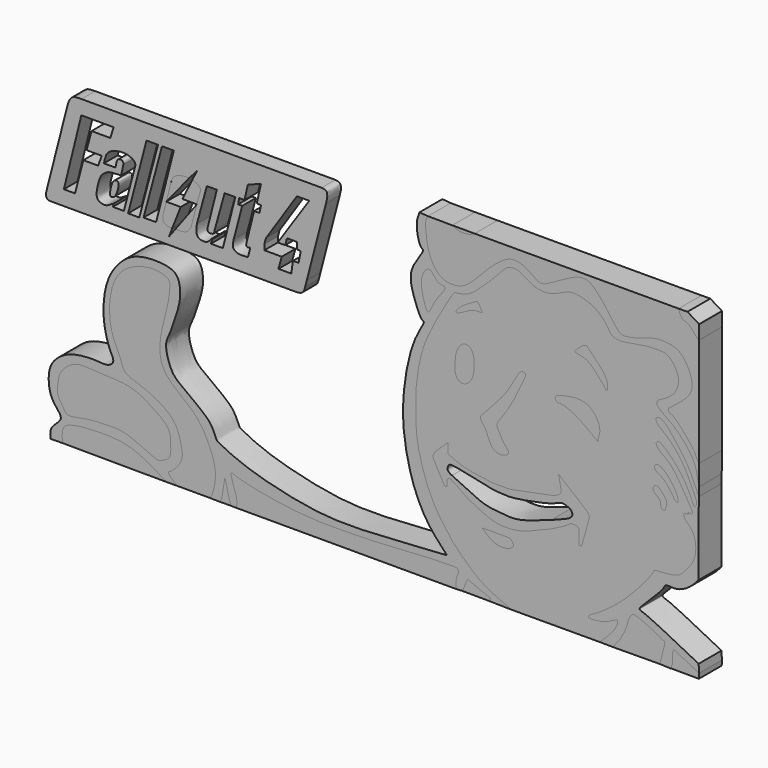
from build123d import *

# Parameters (mm, degrees)
F2_DEPTH       = 3.81
F3_DEPTH       = 50.8
F3_DEPTH_BACK  = 50.8
F4_DEPTH       = 3.81
F7_DEPTH       = 6.35
F8_DEPTH       = 6.35
F9_DEPTH       = 6.35
F10_DEPTH      = 6.35
F11_DEPTH      = 50.8
F11_DEPTH_BACK = 50.8
F12_DEPTH      = 6.35


# Not quite as in the source:
# - the program builds the solid bodies; features that only make, move or delete a surface that nothing else refers to are left out


with BuildPart() as f2:
    # F1 (on Front) → F2 (new body)
    with BuildSketch(Plane.XZ):
        with BuildLine():
            Line((-12.4136926606, 36.7652848363), (-63.8129115105, 36.7652848363))
            add(Edge.make_bspline(
                [(-66.8279528618, 34.8988324404), (-66.5930374758, 35.4970886217), (-66.1023482487, 36.7467209609), (-64.5973817053, 36.7589239674), (-63.8129115105, 36.7652848363)],
                knots=[0, 0, 0, 0, 0.478745758, 1, 1, 1, 1], degree=3))
            Line((-66.8279528618, 34.8988324404), (-71.5658739209, 16.3778848946))
            add(Edge.make_bspline(
                [(-70.5474168062, 14.5114324987), (-70.8911246373, 14.5193117419), (-71.5807384925, 14.5351206203), (-71.7483771612, 15.6377549861), (-71.6249795935, 16.1381857201), (-71.5658739209, 16.3778848946)],
                knots=[0, 0, 0, 0, 0.3411096868, 0.6844009503, 1, 1, 1, 1], degree=3))
            Line((-70.5474168062, 14.5114324987), (-68.8379779458, 14.5114324987))
            Line((-68.8379779458, 14.5114324987), (-17.2951817513, 14.5114324987))
            Line((-17.2951817513, 14.5114324987), (-15.7989468426, 14.5114324987))
            add(Edge.make_bspline(
                [(-14.0476999804, 16.1771159619), (-14.1856649693, 15.6813406422), (-14.4532535126, 14.7197648347), (-15.3598022305, 14.5794182878), (-15.7989468426, 14.5114324987)],
                knots=[0, 0, 0, 0, 0.5155863073, 1, 1, 1, 1], degree=3))
            Line((-14.0476999804, 16.1771159619), (-13.7058505788, 17.5264719874))
            Line((-13.7058505788, 17.5264719874), (-9.3986541033, 34.0373963118))
            add(Edge.make_bspline(
                [(-9.3986541033, 34.0373963118), (-9.2794631114, 34.5027471456), (-9.0568676553, 35.3718143421), (-9.2273719999, 36.6584162884), (-10.0001459599, 36.7299325533), (-10.3821475059, 36.7652848363)],
                knots=[0, 0, 0, 0, 0.3682382464, 0.6877043236, 1, 1, 1, 1], degree=3))
            Line((-10.3821475059, 36.7652848363), (-12.4136926606, 36.7652848363))
        make_face()
    extrude(amount=F2_DEPTH)

    # F0 (on Front) → F3 (cut, two sides)
    with BuildSketch(Plane.XZ) as f3_sk:
        Polygon((-56.6699653864, 33.5655286908), (-63.8487637043, 33.5655286908), (-67.7311718464, 17.8161300719), (-65.2405694127, 17.8161300719), (-63.4092465043, 24.9216724187), (-60.1128563285, 24.9216724187), (-59.3070760369, 27.119262144), (-62.6767128706, 27.119262144), (-61.5779198706, 31.2214307487), (-57.4024952948, 31.2214307487), align=None)
        Polygon((-46.7808097601, 33.3457700908), (-49.3446663022, 33.3457700908), (-53.4468330443, 17.7428778261), (-50.9562306106, 17.7428778261), align=None)
        Polygon((-43.2646647096, 33.3457700908), (-45.9017753601, 33.3457700908), (-50.0039421022, 18.0358905345), (-47.2203269601, 18.0358905345), align=None)
        with BuildLine():
            Line((-33.7026938796, 28.787843883), (-35.9268300235, 28.787843883))
            Line((-35.9268300235, 28.787843883), (-38.1369553506, 20.6729974598))
            add(Edge.make_bspline(
                [(-34.7237996757, 18.7542904168), (-34.7942705526, 18.7755190956), (-35.0111876698, 18.8408633059), (-35.483336033, 17.8389711757), (-37.0910656938, 17.5716890977), (-38.4823420582, 18.4677567251), (-38.2602498605, 19.8857810743), (-38.1369553506, 20.6729974598)],
                knots=[0, 0, 0, 0, 0.0879184805, 0.2706227618, 0.5039064203, 0.7245935905, 1, 1, 1, 1], degree=3))
            Line((-34.7237996757, 18.7542904168), (-35.0293107331, 17.7858132069))
            Line((-35.0293107331, 17.7858132069), (-32.357059703, 17.7858132069))
            Line((-32.357059703, 17.7858132069), (-29.5966751873, 28.6820493639))
            Line((-29.5966751873, 28.6820493639), (-31.9803804159, 28.6820493639))
            Line((-31.9803804159, 28.6820493639), (-34.1977849603, 20.6994023174))
            add(Edge.make_bspline(
                [(-35.7640907168, 20.6507649273), (-35.7779261817, 20.370142077), (-35.805227327, 19.8163966625), (-34.9705905732, 19.7482981395), (-34.3340216083, 19.9094108137), (-34.2448802558, 20.4263121918), (-34.1977849603, 20.6994023174)],
                knots=[0, 0, 0, 0, 0.2567288564, 0.5065960482, 0.7393240705, 1, 1, 1, 1], degree=3))
            Line((-35.7640907168, 20.6507649273), (-33.7026938796, 28.787843883))
        make_face()
        with BuildLine():
            Line((-24.8345918953, 28.9711412042), (-23.8816402853, 33.1264324486))
            Line((-23.8816402853, 33.1264324486), (-26.8109887838, 32.041490078))
            Line((-26.8109887838, 32.041490078), (-27.5433268398, 28.7866592407))
            Line((-27.5433268398, 28.7866592407), (-28.7367645651, 28.7866592407))
            Line((-28.7367645651, 28.7866592407), (-28.9596170187, 27.4700615555))
            Line((-28.9596170187, 27.4700615555), (-28.056461364, 27.4700615555))
            Line((-28.056461364, 27.4700615555), (-29.9493856728, 20.294258371))
            add(Edge.make_bspline(
                [(-29.9493856728, 20.294258371), (-30.092060965, 19.7383291905), (-30.362724298, 18.6836991804), (-29.1729702441, 17.6258337898), (-27.6673140995, 17.7559010596), (-26.7947631998, 17.8312770434)],
                knots=[0, 0, 0, 0, 0.3191430371, 0.6054329153, 1, 1, 1, 1], degree=3))
            Line((-26.7947631998, 17.8312770434), (-26.2655150145, 19.8375806212))
            add(Edge.make_bspline(
                [(-27.0875357091, 20.6291563809), (-27.1541227134, 20.2999555053), (-27.288565148, 19.6352827564), (-26.6086699315, 19.7697251909), (-26.2655150145, 19.8375806212)],
                knots=[0, 0, 0, 0, 0.4952826426, 1, 1, 1, 1], degree=3))
            Line((-27.0875357091, 20.6291563809), (-25.413049385, 27.3271016777))
            Line((-25.413049385, 27.3271016777), (-24.2256876081, 27.3271016777))
            Line((-24.2256876081, 27.3271016777), (-23.8816402853, 28.9711412042))
            Line((-23.8816402853, 28.9711412042), (-24.8345918953, 28.9711412042))
        make_face()
        Polygon((-13.1602361798, 33.3156175911), (-15.8830825239, 33.3156175911), (-22.7770470083, 22.87437208), (-23.1365542859, 21.573740989), (-23.1365542859, 20.3725714236), (-19.269622429, 20.3725714236), (-19.9958086014, 17.7583042532), (-17.1447917819, 17.7583042532), (-16.7751051486, 20.3725714236), (-15.528453514, 20.3725714236), (-15.0296529755, 22.8712726384), (-15.9237217158, 22.8712726384), (-15.9237217158, 24.3749339134), (-18.1182529777, 24.3749339134), (-18.4840094298, 22.8712726384), (-20.1502274722, 22.8712726384), align=None)
        with BuildLine():
            add(Edge.make_bspline(
                [(-56.0185929589, 26.9032054337), (-55.9315318538, 27.1764927811), (-55.7607888192, 27.7124601453), (-54.897529735, 27.8059599362), (-54.4600894732, 27.4133429295), (-54.4765988554, 27.1444736762), (-54.4841401279, 27.0216576755)],
                knots=[0, 0, 0, 0, 0.2903149552, 0.5693616728, 0.8032899767, 1, 1, 1, 1], degree=3))
            Line((-54.4841401279, 27.0216576755), (-54.9910180271, 24.6682912111))
            add(Edge.make_bspline(
                [(-56.6504810475, 18.6222402498), (-56.8782994422, 18.5027217057), (-57.3779649704, 18.2405861723), (-58.3446885415, 17.5424606272), (-59.9100095305, 17.8517225749), (-60.6532111412, 18.8562404414), (-60.1776503547, 21.2198138616), (-59.6312458469, 23.1546101881), (-58.5574681299, 24.0817746184), (-57.404840766, 24.6180593038), (-55.8833951014, 24.6497207495), (-54.9910180271, 24.6682912111)],
                knots=[0, 0, 0, 0, 0.081900036, 0.1796282728, 0.2890494758, 0.3835465603, 0.522869379, 0.6535863473, 0.7573575505, 0.8576823582, 1, 1, 1, 1], degree=3))
            Line((-56.6504810475, 18.6222402498), (-56.8375065923, 17.9108748642))
            Line((-56.8375065923, 17.9108748642), (-54.3889209023, 17.9108748642))
            Line((-54.3889209023, 17.9108748642), (-52.0221553743, 26.9130412489))
            add(Edge.make_bspline(
                [(-58.8288195431, 25.7906652987), (-58.6285272673, 26.6353679225), (-58.2807075766, 28.1022452856), (-57.0637613923, 28.814659604), (-55.5491126764, 29.2714406503), (-53.5448376569, 29.3766637698), (-51.5666326897, 28.3006651858), (-51.8813934139, 27.3418336501), (-52.0221553743, 26.9130412489)],
                knots=[0, 0, 0, 0, 0.1954333106, 0.3393818029, 0.4984152875, 0.6821298917, 0.8578475134, 1, 1, 1, 1], degree=3))
            Line((-58.8288195431, 25.7906652987), (-56.2582165003, 25.7906652987))
            Line((-56.2582165003, 25.7906652987), (-56.0185929589, 26.9032054337))
        make_face()
        with BuildLine():
            add(Edge.make_bspline(
                [(-55.7971820235, 23.2893116772), (-56.007171461, 23.4078330879), (-56.8609223877, 23.1168172963), (-57.1807348709, 21.9058389294), (-57.5572301952, 20.4756311128), (-57.4030916495, 19.5969734365), (-56.5403624052, 19.864360996), (-56.0255461327, 20.5938708576), (-55.5265065234, 22.212219434), (-55.5748715361, 23.1638360681), (-55.7971820235, 23.2893116772)],
                knots=[0, 0, 0, 0, 0.1148834001, 0.2515738645, 0.4032942387, 0.501768148, 0.600291131, 0.715809865, 0.8783758603, 1, 1, 1, 1], degree=3))
        make_face(mode=Mode.SUBTRACT)
        Polygon((-39.8514476016, 29.0725264404), (-44.9494868517, 22.7973349392), (-41.7441688478, 22.7973349392), (-43.6099198481, 18.058598945), (-43.7186323106, 17.7824851125), (-44.3634614513, 16.1313116673), (-42.8970865035, 18.0979792621), (-38.1369553506, 24.4821552187), (-41.3537174463, 24.490237236), (-39.1451600054, 28.9608438894), (-38.1369553506, 31.0016721487), (-39.7662445903, 29.1774030775), align=None)
        with BuildLine():
            Line((-43.8660690067, 26.9905636996), (-44.9494868517, 22.7973349392))
            Line((-44.9494868517, 22.7973349392), (-39.8514476016, 29.0725264404))
            add(Edge.make_bspline(
                [(-43.8660690067, 26.9905636996), (-43.7628166155, 27.3457117417), (-43.564737751, 28.0270259471), (-42.7812553806, 28.5920165781), (-41.9731176873, 28.945427245), (-40.6210563197, 29.1146032025), (-40.082889914, 29.0851800693), (-39.8514476016, 29.0725264404)],
                knots=[0, 0, 0, 0, 0.2077116521, 0.3984729815, 0.5900084539, 0.8236802028, 1, 1, 1, 1], degree=3))
        make_face()
        with BuildLine():
            Line((-41.7441688478, 22.7973349392), (-44.9494868517, 22.7973349392))
            Line((-44.9494868517, 22.7973349392), (-45.6756986678, 19.9451036751))
            add(Edge.make_bspline(
                [(-45.6756986678, 19.9451036751), (-45.7287355556, 19.6003145118), (-45.8359974914, 18.9030120387), (-44.9814559484, 17.9992053131), (-44.0855798465, 18.038000745), (-43.6099198481, 18.058598945)],
                knots=[0, 0, 0, 0, 0.3144948559, 0.6360351894, 1, 1, 1, 1], degree=3))
            Line((-43.6099198481, 18.058598945), (-41.7441688478, 22.7973349392))
        make_face()
        with BuildLine():
            add(Edge.make_bspline(
                [(-37.3789513826, 27.3146970567), (-37.3538073212, 27.4835030951), (-37.3014197079, 27.8352102167), (-37.7396712133, 28.2812787376), (-38.3316934767, 28.7355632037), (-38.8686753494, 28.8842744785), (-39.1451600054, 28.9608438894)],
                knots=[0, 0, 0, 0, 0.2159083302, 0.4498446742, 0.7167325124, 1, 1, 1, 1], degree=3))
            Line((-39.1451600054, 28.9608438894), (-41.3537174463, 24.490237236))
            Line((-41.3537174463, 24.490237236), (-38.1369553506, 24.4821552187))
            Line((-38.1369553506, 24.4821552187), (-37.3789513826, 27.3146970567))
        make_face()
        with BuildLine():
            Line((-38.1369553506, 24.4821552187), (-42.8970865035, 18.0979792621))
            add(Edge.make_bspline(
                [(-39.4998113787, 19.3957794191), (-39.673372729, 19.1869737479), (-40.0151322983, 18.7758146036), (-40.5521962544, 18.1835495656), (-41.8152103185, 18.0861027587), (-42.5416790035, 18.0940777081), (-42.8970865035, 18.0979792621)],
                knots=[0, 0, 0, 0, 0.2288933492, 0.4507137812, 0.7312748013, 1, 1, 1, 1], degree=3))
            Line((-39.4998113787, 19.3957794191), (-38.1369553506, 24.4821552187))
        make_face()
    extrude(amount=-F3_DEPTH, mode=Mode.SUBTRACT)
    extrude(f3_sk.sketch, amount=F3_DEPTH_BACK, mode=Mode.SUBTRACT)

    # F5 (on Front) → F11 (cut, two sides)
    with BuildSketch(Plane.XZ) as f11_sk:
        with BuildLine():
            Line((73.0190351605, 40.6309440732), (71.0514634848, 40.6134128571))
            add(Edge.make_bspline(
                [(71.0514634848, 40.6134128571), (71.1897703074, 40.1407361962), (71.4426160226, 39.2766120258), (72.2686078605, 38.4605475987), (73.256871892, 38.7353609599), (75.2516396689, 35.9107959035), (75.5324992346, 35.9054388501), (75.5949690938, 35.9042473137)],
                knots=[0, 0, 0, 0, 0.2192354105, 0.4007953701, 0.5756499937, 0.905614448, 1, 1, 1, 1], degree=3))
            Line((75.5949690938, 35.9042473137), (75.5949690938, 39.0085279942))
            Line((75.5949690938, 39.0085279942), (75.5122005939, 39.1107201576))
            add(Edge.make_bspline(
                [(73.0190351605, 40.6309440732), (73.850090305, 40.124202768), (74.6811454495, 39.6174614628), (75.5122005939, 39.1107201576)],
                knots=[0, 0, 0, 0, 2.9200949697, 2.9200949697, 2.9200949697, 2.9200949697], degree=3))
        make_face()
    extrude(amount=-F11_DEPTH, mode=Mode.SUBTRACT)
    extrude(f11_sk.sketch, amount=F11_DEPTH_BACK, mode=Mode.SUBTRACT)


with BuildPart() as f4:
    # F0 (on Front) → F4 (new body)
    with BuildSketch(Plane.XZ):
        with BuildLine():
            Line((-43.8660690067, 26.9905636996), (-44.9494868517, 22.7973349392))
            Line((-44.9494868517, 22.7973349392), (-39.8514476016, 29.0725264404))
            add(Edge.make_bspline(
                [(-43.8660690067, 26.9905636996), (-43.7628166155, 27.3457117417), (-43.564737751, 28.0270259471), (-42.7812553806, 28.5920165781), (-41.9731176873, 28.945427245), (-40.6210563197, 29.1146032025), (-40.082889914, 29.0851800693), (-39.8514476016, 29.0725264404)],
                knots=[0, 0, 0, 0, 0.2077116521, 0.3984729815, 0.5900084539, 0.8236802028, 1, 1, 1, 1], degree=3))
        make_face()
    extrude(amount=F4_DEPTH)


with BuildPart() as f4b:
    # F0 (on Front) → F4, piece 2 (new body)
    with BuildSketch(Plane.XZ):
        with BuildLine():
            add(Edge.make_bspline(
                [(-37.3789513826, 27.3146970567), (-37.3538073212, 27.4835030951), (-37.3014197079, 27.8352102167), (-37.7396712133, 28.2812787376), (-38.3316934767, 28.7355632037), (-38.8686753494, 28.8842744785), (-39.1451600054, 28.9608438894)],
                knots=[0, 0, 0, 0, 0.2159083302, 0.4498446742, 0.7167325124, 1, 1, 1, 1], degree=3))
            Line((-39.1451600054, 28.9608438894), (-41.3537174463, 24.490237236))
            Line((-41.3537174463, 24.490237236), (-38.1369553506, 24.4821552187))
            Line((-38.1369553506, 24.4821552187), (-37.3789513826, 27.3146970567))
        make_face()
    extrude(amount=F4_DEPTH)


with BuildPart() as f4c:
    # F0 (on Front) → F4, piece 3 (new body)
    with BuildSketch(Plane.XZ):
        with BuildLine():
            Line((-41.7441688478, 22.7973349392), (-44.9494868517, 22.7973349392))
            Line((-44.9494868517, 22.7973349392), (-45.6756986678, 19.9451036751))
            add(Edge.make_bspline(
                [(-45.6756986678, 19.9451036751), (-45.7287355556, 19.6003145118), (-45.8359974914, 18.9030120387), (-44.9814559484, 17.9992053131), (-44.0855798465, 18.038000745), (-43.6099198481, 18.058598945)],
                knots=[0, 0, 0, 0, 0.3144948559, 0.6360351894, 1, 1, 1, 1], degree=3))
            Line((-43.6099198481, 18.058598945), (-41.7441688478, 22.7973349392))
        make_face()
    extrude(amount=F4_DEPTH)


with BuildPart() as f4d:
    # F0 (on Front) → F4, piece 4 (new body)
    with BuildSketch(Plane.XZ):
        with BuildLine():
            Line((-38.1369553506, 24.4821552187), (-42.8970865035, 18.0979792621))
            add(Edge.make_bspline(
                [(-39.4998113787, 19.3957794191), (-39.673372729, 19.1869737479), (-40.0151322983, 18.7758146036), (-40.5521962544, 18.1835495656), (-41.8152103185, 18.0861027587), (-42.5416790035, 18.0940777081), (-42.8970865035, 18.0979792621)],
                knots=[0, 0, 0, 0, 0.2288933492, 0.4507137812, 0.7312748013, 1, 1, 1, 1], degree=3))
            Line((-39.4998113787, 19.3957794191), (-38.1369553506, 24.4821552187))
        make_face()
    extrude(amount=F4_DEPTH)


with BuildPart() as f7:
    # F5 (on Front) → F7 (new body)
    with BuildSketch(Plane.XZ):
        with BuildLine():
            add(Edge.make_bspline(
                [(-40.6401716173, -30.3776804358), (-41.5448572577, -29.5201807357), (-42.8205399649, -28.3110341661), (-41.9079778037, -28.1649947451), (-38.9262008276, -25.2690898767), (-39.6425750234, -21.9207413573), (-40.7729732105, -17.0739514623), (-47.9495227407, -13.3058290183), (-52.5089788791, -12.3014132072), (-52.960088641, -9.2910364738), (-55.3492706294, -5.532379551), (-55.8872939809, 1.6360287505), (-53.8209779608, 7.3796636694), (-49.6946606264, 9.8562396668), (-45.4784942254, 10.6737999753), (-42.3385991044, 9.7288203685), (-41.8739940796, 8.1751631117), (-43.0510242174, 1.7933695088), (-44.2813052857, -1.7012085278), (-44.6569854103, -8.2517046927), (-40.1960798652, -12.0304985003), (-35.705923736, -15.4357495082), (-33.2382097555, -20.1392578583), (-31.4508960164, -25.0285737622), (-32.5529036806, -29.468786726), (-33.0174558134, -30.1121119274), (-33.1186040792, -30.2274059699)],
                knots=[0, 0, 0, 0, 0.0341427126, 0.0481440912, 0.0882914037, 0.1258609665, 0.1706120303, 0.2290606102, 0.2719927927, 0.3047170201, 0.348065628, 0.4034481482, 0.4536414825, 0.4977618465, 0.540996773, 0.5760398354, 0.6001823779, 0.6517776708, 0.6943955894, 0.7445158309, 0.7934040004, 0.8425564368, 0.8898049476, 0.9378769585, 0.9816349027, 0.9941308196, 0.9941308196, 0.9941308196, 0.9941308196], degree=3))
            Line((-40.6401716173, -30.3776804358), (-33.2602262497, -30.3776804358))
            add(Edge.make_bspline(
                [(-33.1186040792, -30.2274059699), (-33.1661121912, -30.2815581813), (-33.2131692204, -30.3296193085), (-33.2602262497, -30.3776804358)],
                knots=[0.9941308196, 0.9941308196, 0.9941308196, 0.9941308196, 1, 1, 1, 1], degree=3))
        make_face()
    extrude(amount=F7_DEPTH)


with BuildPart() as f7b:
    # F5 (on Front) → F7, piece 2 (new body)
    with BuildSketch(Plane.XZ):
        with BuildLine():
            add(Edge.make_bspline(
                [(-64.9122595787, -24.3510659784), (-64.0944023238, -24.6359030412), (-60.5483775248, -23.6357743738), (-56.3503770691, -23.5568357937), (-51.882756585, -23.2562107688), (-45.1274480755, -26.9945507012), (-44.0736520456, -26.5594564533), (-41.7712103095, -25.6234051097), (-41.9867580107, -22.6867987207), (-41.9238346863, -19.614624778), (-45.7571879989, -16.9597427911), (-50.7096471608, -13.7612227916), (-58.2178745804, -14.1337228072), (-63.3034354416, -13.1049472656), (-66.9452489043, -16.7076397996), (-66.8643823483, -18.7979608226), (-67.4922258789, -21.0642115513), (-65.7629013645, -23.1510353399), (-65.3978736062, -24.181940043), (-64.9122595787, -24.3510659784)],
                knots=[0, 0, 0, 0, 0.0636241215, 0.1289358926, 0.1968620529, 0.2805863176, 0.3128439435, 0.3574753263, 0.408547408, 0.4614235174, 0.5258525697, 0.6018874424, 0.6867686733, 0.7570713816, 0.822126869, 0.8663924789, 0.9121945158, 0.9622223002, 1, 1, 1, 1], degree=3))
        make_face()
    extrude(amount=F7_DEPTH)


with BuildPart() as f7c:
    # F5 (on Front) → F7, piece 3 (new body)
    with BuildSketch(Plane.XZ):
        with BuildLine():
            add(Edge.make_bspline(
                [(-66.0086646676, -30.2900373936), (-66.0843713987, -29.2458909348), (-66.2216891642, -27.3520057225), (-64.4478774808, -25.8813400443), (-57.7499710133, -25.3831622164), (-50.5056460942, -25.6090327706), (-45.461129337, -28.7533449571), (-42.8219400346, -30.3983855993)],
                knots=[0, 0, 0, 0, 0.1483911377, 0.2691536029, 0.4940587683, 0.7353017642, 1, 1, 1, 1], degree=3))
            Line((-66.0086646676, -30.2900373936), (-42.8219400346, -30.3983855993))
        make_face()
    extrude(amount=F7_DEPTH)


with BuildPart() as f7d:
    # F5 (on Front) → F7, piece 4 (new body)
    with BuildSketch(Plane.XZ):
        with BuildLine():
            Line((75.5356550217, 5.2311006002), (75.5660608411, 7.1465815417))
            add(Edge.make_bspline(
                [(75.1312151551, 9.5434607938), (75.2761637171, 8.7445010431), (75.4211122791, 7.9455412924), (75.5660608411, 7.1465815417)],
                knots=[0, 0, 0, 0, 2.4360051148, 2.4360051148, 2.4360051148, 2.4360051148], degree=3))
            add(Edge.make_bspline(
                [(20.8272319287, -21.4312896132), (19.7081994534, -19.9845242585), (17.4087878834, -17.0116802444), (14.6780433437, -11.606074421), (12.6218569894, -4.0043270402), (12.580405615, 1.5447490505), (12.5533584201, 5.9481195507), (13.2105439686, 10.8732285471), (14.6599862079, 16.6434933744), (19.6765021047, 25.4118760109), (21.2322025325, 27.7306524367), (21.5668913033, 27.5411162655), (24.2103933068, 27.9979705456), (26.7293114506, 30.0258597357), (30.6994992812, 33.9009430526), (33.0176624045, 36.82234819), (36.0044520904, 36.55891581), (39.1342351997, 33.8723824832), (43.2396715716, 34.2117170054), (45.9872870654, 35.853238569), (47.9339639056, 36.2214419835), (51.8809553526, 35.3776550628), (54.9559521045, 32.6503171749), (55.8284738998, 30.5792890326), (58.0594823949, 29.7314985443), (62.9606191955, 31.0327255685), (66.1685335067, 31.0455861895), (68.5919551624, 31.0559496147), (70.3159785764, 29.0379266043), (71.2485346961, 26.9370500832), (70.7938207938, 24.2532050476), (68.3382606046, 21.9558162024), (65.9386382123, 21.1750781063), (66.467512556, 19.4466160477), (70.5111689003, 17.3468166476), (74.5907574875, 12.1942251311), (74.9815140249, 10.2776948348), (75.1312151551, 9.5434607938)],
                knots=[0, 0, 0, 0, 0.0355058038, 0.0729580756, 0.1154432611, 0.1511430706, 0.1826231394, 0.2155513942, 0.2535583828, 0.3024747043, 0.324968185, 0.332200497, 0.3553429618, 0.3835908655, 0.4195705938, 0.4479809573, 0.4719856798, 0.5021729478, 0.5321715334, 0.558769165, 0.5796286856, 0.6095998689, 0.6401984318, 0.6619487718, 0.6836987638, 0.7177154711, 0.7454548913, 0.7679405287, 0.7916510994, 0.8143832434, 0.8383938948, 0.8662640615, 0.8884779963, 0.9045651974, 0.9368783559, 0.9758177265, 1, 1, 1, 1], degree=3))
            add(Edge.make_bspline(
                [(33.9054688811, -30.4471217096), (32.4717566495, -29.86673205), (29.552345146, -28.6849075447), (25.2676003286, -26.0123972641), (22.3685331271, -23.0214429691), (20.8272319287, -21.4312896132)],
                knots=[0, 0, 0, 0, 0.311274671, 0.6338362993, 1, 1, 1, 1], degree=3))
            Line((33.9054688811, -30.4471217096), (53.5158663988, -30.3929466754))
            add(Edge.make_bspline(
                [(51.3550490141, -25.7696639746), (51.1556198321, -25.9532370321), (50.7885926867, -26.2910827505), (51.5200567731, -26.6348703816), (55.3222891872, -26.1938205266), (57.7390388246, -24.1817729611), (57.3128592995, -26.7267190358), (55.0408498878, -28.9204823428), (53.5158663988, -30.3929466754)],
                knots=[0, 0, 0, 0, 0.0935685364, 0.1722024453, 0.4079909545, 0.5854859823, 0.721776226, 1, 1, 1, 1], degree=3))
            add(Edge.make_bspline(
                [(73.8960281014, -8.5379499942), (73.3842030209, -9.1639029203), (72.3442496025, -10.4357473648), (70.8480130069, -12.2470675485), (65.5102046469, -12.2365017361), (65.7400922316, -12.6688080897), (61.37368792, -18.3414675152), (55.261644707, -23.5585978933), (52.4882645901, -25.1282834173), (51.3550490141, -25.7696639746)],
                knots=[0, 0, 0, 0, 0.1157705032, 0.2352286652, 0.398542399, 0.4288229108, 0.6198829879, 0.8446824811, 1, 1, 1, 1], degree=3))
            add(Edge.make_bspline(
                [(75.5356550217, 5.2311006002), (74.7626647836, 7.1228799176), (73.2678596313, 10.7811945138), (70.0822554368, 14.7100878486), (67.7758981117, 17.914694897), (65.9680947546, 17.8893744506), (66.0113776537, 16.4799861555), (68.607824424, 14.9249334205), (72.4018200734, 10.5314985275), (74.1527949444, 6.0545440277), (75.0551531455, 4.4737041799), (75.0959911288, 3.487784065), (74.5123219401, 2.6135371331), (73.9430376257, 4.2994157353), (72.3040835165, 7.7696795478), (69.4258345891, 11.0919736188), (67.4508908226, 12.8277162592), (66.608690224, 13.2313084997), (65.8074287998, 12.753801722), (66.6757295739, 11.2599536118), (69.0776545078, 9.9344461082), (71.1158982827, 7.0917845588), (73.6038771059, 2.7715316582), (74.0375351628, 2.08154199), (74.2818580241, 1.1185256883), (72.848402942, 1.5482462823), (73.5413937853, 0.8420566092), (71.9837611338, 1.242304762), (72.3197400052, -0.273803786), (74.0724763196, -1.4855886575), (74.8804037246, -3.7062050245), (74.9526529218, -6.560679357), (74.2342389311, -7.9050533124), (73.8960281014, -8.5379499942)],
                knots=[0, 0, 0, 0, 0.0546071505, 0.1055990695, 0.1488532775, 0.1734404601, 0.1943756762, 0.2318182713, 0.2866219548, 0.3356728218, 0.3647267841, 0.386371868, 0.4039624049, 0.4282243253, 0.4731797836, 0.5210054282, 0.5565571003, 0.5765962244, 0.5939819613, 0.6199797098, 0.6565998764, 0.6999476244, 0.7489869416, 0.7700150766, 0.7870050312, 0.8078045028, 0.820129388, 0.8413638274, 0.8631501506, 0.8958649439, 0.9298197866, 0.9669609605, 1, 1, 1, 1], degree=3))
        make_face()
        with BuildLine():
            add(Edge.make_bspline(
                [(27.3189861327, -16.5305063128), (27.4507137947, -16.6559205314), (27.8491965195, -17.035304776), (29.9718454437, -18.935274575), (33.1560824896, -19.0188222048), (34.7603123168, -17.6238924087), (33.8879159465, -16.889937268), (33.4606878459, -16.5305063128)],
                knots=[0, 0, 0, 0, 0.1227042334, 0.3711864047, 0.6385688676, 0.8230007122, 1, 1, 1, 1], degree=3))
            Line((27.3189861327, -16.5305063128), (33.4606878459, -16.5305063128))
        make_face(mode=Mode.SUBTRACT)
        with BuildLine():
            add(Edge.make_bspline(
                [(29.5570250601, -6.9518866949), (28.5054109283, -6.8348146507), (26.3221292586, -6.591758533), (22.5925894251, -5.8620742549), (20.6374024114, -4.9372962484), (19.7016131133, -4.4946800917)],
                knots=[0, 0, 0, 0, 0.3263720735, 0.6775889978, 1, 1, 1, 1], degree=3))
            add(Edge.make_bspline(
                [(29.5570250601, -6.9518866949), (30.8705219904, -7.0168720697), (33.6334599434, -7.1535686652), (37.8066471876, -5.9883978013), (44.4948092514, -5.0762858825), (44.8480898406, -3.8993501363), (44.9562259018, -3.5391005222)],
                knots=[0, 0, 0, 0, 0.2539536733, 0.5341910027, 0.8574199891, 1, 1, 1, 1], degree=3))
            Line((44.9562259018, -3.5391005222), (44.3410947919, -0.4880409106))
            Line((44.3410947919, -0.4880409106), (50.2177216113, -5.3168945014))
            add(Edge.make_bspline(
                [(50.2177216113, -5.3168945014), (50.6102232429, -5.632318237), (51.3559777106, -6.2316244336), (51.1400131135, -7.0328879201), (51.0377138853, -7.4124345556)],
                knots=[0, 0, 0, 0, 0.5263148242, 1, 1, 1, 1], degree=3))
            Line((51.0377138853, -7.4124345556), (49.4888350368, -12.9246162251))
            add(Edge.make_bspline(
                [(49.4888350368, -12.9246162251), (49.2819870512, -12.9246162251), (49.0751390656, -12.9246162251), (48.86829108, -12.9246162251)],
                knots=[0, 0, 0, 0, 0.6205439568, 0.6205439568, 0.6205439568, 0.6205439568], degree=3))
            Line((48.86829108, -12.9246162251), (48.86829108, -10.0170345977))
            add(Edge.make_bspline(
                [(48.86829108, -10.0170345977), (48.8615206278, -9.7854080417), (48.8443878118, -9.1992706554), (47.0565315084, -9.2480214449), (47.0133140651, -9.3316671533), (45.4115455704, -10.4479907172), (43.8341803737, -11.2103733672), (42.9326407611, -11.6461114958)],
                knots=[0, 0, 0, 0, 0.1493110148, 0.3778356398, 0.4387442369, 0.6792155017, 1, 1, 1, 1], degree=3))
            add(Edge.make_bspline(
                [(42.9326407611, -11.6461114958), (41.923505909, -12.0844370405), (39.7356611691, -13.0347443608), (35.4392586983, -14.769811641), (30.9012542238, -14.8221307532), (29.1846642419, -14.2023430155), (28.448369354, -13.9364982024)],
                knots=[0, 0, 0, 0, 0.2403478181, 0.5210836872, 0.7945789987, 1, 1, 1, 1], degree=3))
            add(Edge.make_bspline(
                [(28.448369354, -13.9364982024), (26.8111187618, -13.2027729312), (23.9546696089, -11.9226702156), (21.6804262437, -9.9987717931), (20.7735378854, -9.6365362826), (20.3687022635, -9.1420897408), (19.6250521066, -9.3375964532), (19.4905479923, -9.9756983435), (19.6648026906, -11.2406917298), (19.1408387638, -11.0308439987), (18.9165342599, -10.9410099685)],
                knots=[0, 0, 0, 0, 0.2523202857, 0.4402136544, 0.5458241391, 0.6289633219, 0.7151469196, 0.8050624297, 0.916548883, 1, 1, 1, 1], degree=3))
            Line((18.9165342599, -10.9410099685), (16.7929157615, -7.0316195488))
            add(Edge.make_bspline(
                [(16.7929157615, -7.0316195488), (16.6496159091, -6.8017204049), (16.3723115228, -6.3568348035), (16.4746378505, -5.6238488624), (16.7790534866, -5.2065114312), (16.9365629554, -4.9905744381)],
                knots=[0, 0, 0, 0, 0.3403950463, 0.6587099558, 1, 1, 1, 1], degree=3))
            Line((16.9365629554, -4.9905744381), (19.7712983936, -2.2707614116))
            Line((19.7712983936, -2.2707614116), (19.7016131133, -4.4946800917))
        make_face(mode=Mode.SUBTRACT)
        with BuildLine():
            add(Edge.make_bspline(
                [(65.3686448932, 3.2193842344), (65.5491112547, 2.7016566813), (67.240201664, 2.0103883933), (66.8727236991, 0.5191407051), (68.0409292848, -0.3736098854), (68.3215358571, 1.1185536394), (68.6219143553, 2.1872299696), (66.6902188951, 4.2656725595), (65.7513738019, 4.4548981905), (65.2346992015, 3.6036518321), (65.3686448932, 3.2193842344)],
                knots=[0, 0, 0, 0, 0.1540468511, 0.2799967621, 0.3823696091, 0.4956795554, 0.6125107114, 0.7884001066, 0.8856633899, 1, 1, 1, 1], degree=3))
        make_face(mode=Mode.SUBTRACT)
        with BuildLine():
            add(Edge.make_bspline(
                [(36.1209399998, 16.92520082), (35.4456308538, 16.5879956251), (33.8751094283, 13.3416726335), (31.724812132, 10.2553680795), (27.4751921427, 5.8005581423), (26.6368600912, 4.8476536817), (28.4308885879, 2.9961396275), (29.143770564, -0.2711749657), (31.5541350127, -1.178285934), (33.8255164091, -0.0523947903), (32.1895692887, 1.3185206899), (31.0743038737, 3.6967926568), (30.4630487355, 4.6673167865), (31.0681279003, 5.6948647682), (33.7015267158, 9.24207421), (35.9005618289, 13.8724796169), (37.0283168237, 16.0648428287), (36.9626665337, 16.9076109675), (36.4174564839, 17.0732617479), (36.1209399998, 16.92520082)],
                knots=[0, 0, 0, 0, 0.0744714076, 0.1559889596, 0.2492763984, 0.2861424977, 0.3430246926, 0.412639342, 0.4704416692, 0.5211466051, 0.5690541016, 0.6329607134, 0.6711264919, 0.7084330058, 0.7888501922, 0.8786232481, 0.9368157745, 0.967300902, 1, 1, 1, 1], degree=3))
        make_face(mode=Mode.SUBTRACT)
        with BuildLine():
            add(Edge.make_bspline(
                [(22.9565948248, 18.0230028927), (22.5922138055, 17.7666357148), (21.5722571805, 16.5698137351), (21.2759437623, 14.0882049406), (21.2252454984, 10.9972027449), (23.2483114546, 9.9131899997), (25.2230499422, 11.5429280072), (25.6892885891, 14.3342934889), (25.5135014403, 16.8321688996), (24.6356982611, 18.1414804253), (23.585054307, 18.2879504005), (23.1801344304, 18.1802784225), (22.9565948248, 18.0230028927)],
                knots=[0, 0, 0, 0, 0.0981672345, 0.216638811, 0.3410486155, 0.4366262099, 0.5437202471, 0.6667336506, 0.7823848017, 0.8694083856, 0.9397765972, 1, 1, 1, 1], degree=3))
        make_face(mode=Mode.SUBTRACT)
        with BuildLine():
            add(Edge.make_bspline(
                [(43.5981042683, 14.33346048), (43.5226760533, 14.0377591166), (44.0128248448, 13.2972985384), (45.0734277985, 13.7194945938), (49.2425503452, 11.8984364099), (53.336555704, 8.4528124709), (52.9314822476, 8.9584759644), (53.9581021084, 10.9359697655), (52.7381448404, 13.8520248211), (50.1463341118, 15.9632015248), (45.9655763314, 15.4521401203), (43.7190922888, 14.8077700286), (43.5981042683, 14.33346048)],
                knots=[0, 0, 0, 0, 0.0629790853, 0.1247119392, 0.271715009, 0.4132987085, 0.4373895232, 0.5297772784, 0.6453357007, 0.7615939215, 0.8989805757, 1, 1, 1, 1], degree=3))
        make_face(mode=Mode.SUBTRACT)
        with BuildLine():
            add(Edge.make_bspline(
                [(68.0600628257, 5.7594329119), (68.3467198844, 5.4457751869), (69.3768165389, 4.4142430538), (70.3286032662, 2.4444304976), (70.9387000241, 2.4739083426), (70.9737674725, 3.726761442), (69.4233667463, 6.3963889802), (67.2829826077, 8.5000175302), (65.8940726244, 8.6614575332), (65.4090263901, 7.2748993818), (67.625363691, 6.2832567818), (67.8828473631, 5.9533405696), (68.0600628257, 5.7594329119)],
                knots=[0, 0, 0, 0, 0.1131196564, 0.2323104411, 0.2782457798, 0.3578259707, 0.504329956, 0.6470253057, 0.7313328172, 0.8106009302, 0.9300678228, 1, 1, 1, 1], degree=3))
        make_face(mode=Mode.SUBTRACT)
        with BuildLine():
            add(Edge.make_bspline(
                [(26.2823738158, 27.3888073862), (26.6160251495, 27.1630574748), (27.3544276129, 25.7533423842), (27.4055011882, 25.4736904913), (25.1067163492, 25.8777257774), (22.1188642489, 23.556296946), (21.260183266, 23.9156935087), (23.1276081869, 25.9209103809), (25.7506327715, 27.114925547), (26.1151773751, 27.5019332089), (26.2823738158, 27.3888073862)],
                knots=[0, 0, 0, 0, 0.1443612772, 0.1822780442, 0.3269282617, 0.5274088581, 0.5896268962, 0.7467419734, 0.9276589383, 1, 1, 1, 1], degree=3))
        make_face(mode=Mode.SUBTRACT)
        with BuildLine():
            add(Edge.make_bspline(
                [(48.1272526085, 24.9930359423), (48.5704481434, 25.4387492041), (50.3365532664, 27.1933677533), (51.2461786046, 25.8547611865), (55.7249847092, 21.9660329777), (55.1708490361, 18.9188514904), (54.6007013422, 19.9808408524), (52.4542839155, 22.4357993285), (50.5112830719, 24.2924356605), (47.6864305994, 24.5437043411), (47.9647811297, 24.8296414875), (48.1272526085, 24.9930359423)],
                knots=[0, 0, 0, 0, 0.1255873944, 0.2100683019, 0.3987159844, 0.5075344349, 0.5664492301, 0.7063043201, 0.8400869812, 0.9539607959, 1, 1, 1, 1], degree=3))
        make_face(mode=Mode.SUBTRACT)
    extrude(amount=F7_DEPTH)


with BuildPart() as f7e:
    # F5 (on Front) → F7, piece 5 (new body)
    with BuildSketch(Plane.XZ):
        with BuildLine():
            add(Edge.make_bspline(
                [(-31.1588550476, -30.4149316569), (-30.9723264984, -30.3076727016), (-30.2900879915, -29.6346589757), (-29.9893918917, -23.7638473088), (-29.3695458137, -27.7626908208), (-28.8457794217, -29.4413103598), (-28.549592942, -30.3905587643)],
                knots=[0.0509120537, 0.0509120537, 0.0509120537, 0.0509120537, 0.1664855302, 0.4971991425, 0.7156693934, 1, 1, 1, 1], degree=3))
            Line((-31.1588550476, -30.4149316569), (-28.549592942, -30.3905587643))
        make_face()
    extrude(amount=F7_DEPTH)


with BuildPart() as f8:
    # F5 (on Front) → F8 (new body)
    with BuildSketch(Plane.XZ):
        with BuildLine():
            add(Edge.make_bspline(
                [(-27.418313548, -30.4093882442), (-27.2581694745, -29.9885277025), (-26.8273156242, -28.8562386279), (-29.2441063342, -23.2477513315), (-26.6469105461, -24.8466260386), (-11.24565601, -27.6863999046), (0.3083461602, -26.890392548), (3.7454153174, -27.1538467651), (21.6939009938, -25.7339766911), (21.7785764184, -26.3907132845), (22.392655475, -26.6312330754), (21.369204686, -28.3956677359), (21.4931598753, -29.707671933), (21.5583425015, -30.3975977004)],
                knots=[0, 0, 0, 0, 0.0586567262, 0.1578108749, 0.2073600604, 0.3880269603, 0.5397780854, 0.638117008, 0.8222635908, 0.8480324651, 0.8759854391, 0.9347861529, 1, 1, 1, 1], degree=3))
            Line((-27.418313548, -30.4093882442), (21.5583425015, -30.3975977004))
        make_face()
    extrude(amount=F8_DEPTH)


with BuildPart() as f8b:
    # F5 (on Front) → F8, piece 2 (new body)
    with BuildSketch(Plane.XZ):
        with BuildLine():
            Line((75.5608379841, -30.4237548262), (75.6070837379, -29.3107386678))
            add(Edge.make_bspline(
                [(75.6070837379, -29.3107386678), (73.0541891168, -27.988257658), (70.2080752308, -26.513879697), (70.0268464932, -26.4823635179), (69.5135094199, -27.3251234587), (69.8555243839, -29.3093558773), (69.4704623217, -30.0788315071), (69.3029556228, -30.3958489047)],
                knots=[0, 0, 0, 0, 0.4002898621, 0.4462661817, 0.5905496951, 0.822735502, 0.9909261541, 0.9909261541, 0.9909261541, 0.9909261541], degree=3))
            Line((69.3029556228, -30.3958489047), (75.5608379841, -30.4237548262))
        make_face()
    extrude(amount=F8_DEPTH)


with BuildPart() as f9:
    # F5 (on Front) → F9 (new body)
    with BuildSketch(Plane.XZ):
        with BuildLine():
            add(Edge.make_bspline(
                [(22.9860711843, -30.3192865103), (23.4293986197, -29.1386590036), (24.0742936467, -27.4212358372), (24.6182531323, -28.023821572), (29.1943736757, -29.6416112956), (29.1849857494, -29.8030381569), (29.0803191881, -30.129793839), (29.0058478713, -30.362283811)],
                knots=[0, 0, 0, 0, 0.2946440862, 0.4286098508, 0.8117162886, 0.8660342354, 1, 1, 1, 1], degree=3))
            Line((22.9860711843, -30.3192865103), (29.0058478713, -30.362283811))
        make_face()
    extrude(amount=F9_DEPTH)


with BuildPart() as f9b:
    # F5 (on Front) → F9, piece 2 (new body)
    with BuildSketch(Plane.XZ):
        with BuildLine():
            add(Edge.make_bspline(
                [(66.8956339359, -30.3471405059), (67.3680910027, -28.3087485437), (67.9373304311, -25.8527940095), (68.1923140691, -25.5643603135), (61.0347512099, -21.9619823817), (60.7059243749, -22.8291698511), (59.8812746054, -23.4772267392), (59.6637990793, -25.4206498807), (58.213135821, -28.3042817634), (56.9646800867, -29.7330524058), (56.3611462712, -30.4237548262)],
                knots=[0, 0, 0, 0, 0.1812113304, 0.2183322917, 0.4476872877, 0.5127254425, 0.5922993526, 0.7074207023, 0.8585600634, 1, 1, 1, 1], degree=3))
            Line((56.3611462712, -30.4237548262), (66.8956339359, -30.3471405059))
        make_face()
    extrude(amount=F9_DEPTH)


with BuildPart() as f10:
    # F5 (on Front) → F10 (new body)
    with BuildSketch(Plane.XZ):
        with BuildLine():
            add(Edge.make_bspline(
                [(19.0748684108, 27.8386455029), (19.2909115361, 27.3910090777), (16.6019677292, 24.8492457561), (15.3442438917, 20.3453528143), (13.9959753226, 25.0257710023), (13.510948136, 27.889127158), (15.1608199003, 30.806457747), (16.617543205, 29.5899020952), (17.3867660493, 27.9946451333), (18.9430672665, 28.111734466), (19.0748684108, 27.8386455029)],
                knots=[0, 0, 0, 0, 0.1556052047, 0.2973434118, 0.4354222126, 0.5829076405, 0.7081297852, 0.7992495601, 0.9050701381, 1, 1, 1, 1], degree=3))
        make_face()
    extrude(amount=F10_DEPTH)


with BuildPart() as f10b:
    # F5 (on Front) → F10, piece 2 (new body)
    with BuildSketch(Plane.XZ):
        with BuildLine():
            Line((20.7139514387, 40.5474938452), (15.2710275725, 40.5757389963))
            add(Edge.make_bspline(
                [(15.2710275725, 40.5757389963), (15.0972865219, 40.2928314671), (14.6172548149, 39.511182089), (14.9340769002, 35.9166255451), (15.7280601483, 32.4571482557), (17.5999068093, 29.7706026151), (19.8705849708, 28.8071641802), (23.615428331, 29.126651268), (27.1030000473, 33.115273254), (30.3047206014, 36.2190193056), (32.8252582479, 37.9684059655), (34.6394463119, 38.3984465855), (37.0322720672, 37.8278179766), (39.6995747867, 35.5488626846), (41.4468127352, 35.5921833964), (45.9752105789, 38.4199161269), (49.3299696217, 39.9368341223), (51.6579514603, 39.3746262045), (53.1874658082, 37.6212668414), (54.0600381792, 36.6209931672)],
                knots=[0, 0, 0, 0, 0.0356532785, 0.098506968, 0.1639112514, 0.2229938152, 0.2742117466, 0.3364398615, 0.4135105707, 0.4861553311, 0.5439029158, 0.5881701926, 0.6406363287, 0.7022600635, 0.7445465221, 0.8220944674, 0.8871839473, 0.93563959, 1, 1, 1, 1], degree=3))
            add(Edge.make_bspline(
                [(54.0600381792, 36.6209931672), (55.7508939716, 34.2670079353), (57.7681390794, 31.4586281704), (58.2330044962, 31.6211480629), (58.6834906373, 31.0520221727), (62.994765494, 32.1072576208), (65.7669841593, 33.219426954), (68.1437807635, 33.1827405546), (71.3644571543, 32.7731323479), (73.6383454686, 29.1956401275), (74.4346876202, 25.8683887336), (72.6299532577, 23.2078065172), (68.9181382197, 20.3993369541), (68.7265812209, 20.3609684593), (68.8459365815, 19.4696885673), (69.9234045664, 19.5494068167), (74.2709131584, 14.5432920621), (74.8338315902, 13.1529935966), (75.0397890806, 12.6443188637)],
                knots=[0, 0, 0, 0, 0.1024771565, 0.1222585294, 0.1500478149, 0.2333340761, 0.3067681333, 0.3678418106, 0.4383705529, 0.5200515029, 0.5921387735, 0.6666896049, 0.7515672428, 0.7665914315, 0.7992217984, 0.8374975959, 0.9405445168, 1, 1, 1, 1], degree=3))
            add(Edge.make_bspline(
                [(75.0397890806, 12.6443188637), (75.224849085, 12.3504089812), (75.4099090894, 12.0564990987), (75.5949690938, 11.7625892162)],
                knots=[0, 0, 0, 0, 1.041955862, 1.041955862, 1.041955862, 1.041955862], degree=3))
            Line((75.5949690938, 11.7625892162), (75.5949690938, 35.9042473137))
            add(Edge.make_bspline(
                [(71.0514634848, 40.6134128571), (71.1897703074, 40.1407361962), (71.4426160226, 39.2766120258), (72.2686078605, 38.4605475987), (73.256871892, 38.7353609599), (75.2516396689, 35.9107959035), (75.5324992346, 35.9054388501), (75.5949690938, 35.9042473137)],
                knots=[0, 0, 0, 0, 0.2192354105, 0.4007953701, 0.5756499937, 0.905614448, 1, 1, 1, 1], degree=3))
            Line((71.0514634848, 40.6134128571), (25.6746616215, 40.5474938452))
            add(Edge.make_bspline(
                [(20.7139514387, 40.5474938452), (21.1311136188, 40.3194856954), (22.0520586447, 39.8161251766), (24.3365526427, 39.8161253578), (25.2574987989, 40.3194857029), (25.6746616215, 40.5474938452)],
                knots=[0, 0, 0, 0, 0.311755369, 0.6882444528, 1, 1, 1, 1], degree=3))
        make_face()
    extrude(amount=F10_DEPTH)


with BuildPart() as f12:
    # F5 (on Front) → F12 (new body)
    with BuildSketch(Plane.XZ):
        with BuildLine():
            add(Edge.make_bspline(
                [(-68.6843767762, -30.3366594017), (-68.7538686656, -29.5094820926), (-68.9013049327, -27.7545156403), (-65.2539951533, -25.6495089376), (-68.3715594537, -23.0562910544), (-69.2375001479, -19.6209153267), (-68.9645346105, -15.9633031666), (-66.9513270398, -13.6593393985), (-64.101991977, -12.0074977982), (-59.0973716913, -11.4573503278), (-55.9434054169, -12.0684716176), (-54.2904033392, -10.6753249532), (-55.5032182329, -8.7315426058), (-56.4719536362, -5.6596752737), (-57.0588239866, -1.9371995787), (-56.6171733877, 3.8987836422), (-54.2818961971, 8.3855221173), (-50.7682207634, 11.5202132287), (-46.2150180657, 12.3883643414), (-40.9134247308, 11.9036021437), (-39.837239243, 9.2801219955), (-39.7224289236, 6.2252549476), (-40.7862928763, 2.6688856282), (-42.0489395331, -1.1094884648), (-43.4856047583, -3.4563715242), (-41.8438065399, -8.6347588361), (-39.7720999003, -10.3326692596), (-35.505871144, -13.4174963419), (-32.7506454192, -15.7393197373), (-31.7676218353, -18.5755699275), (-31.389550492, -18.8954097941), (-26.2480426808, -21.4995465338), (-17.2020020298, -23.9883968883), (-8.2269460501, -25.6421163152), (0.9801082403, -25.7475331524), (12.9670110804, -24.856779063), (17.571422362, -24.5785343105), (19.5202827454, -24.4607646018)],
                knots=[0, 0, 0, 0, 0.0220691412, 0.0468226123, 0.0712931346, 0.0983848421, 0.1249016124, 0.1487980695, 0.174340457, 0.2061826373, 0.2314156734, 0.2488894525, 0.2686302327, 0.2941154742, 0.3218074782, 0.3558186823, 0.3876051736, 0.4174193731, 0.4481894489, 0.4794818267, 0.5013689386, 0.5257816886, 0.5533888806, 0.5814269525, 0.6046459475, 0.6359795431, 0.6597827191, 0.6918287059, 0.7198332256, 0.7427164512, 0.7520512856, 0.7839877576, 0.828870816, 0.871453087, 0.914927517, 0.9639922714, 1, 1, 1, 1], degree=3))
            Line((-68.6843767762, -30.3366594017), (-66.0086646676, -30.2900373936))
            add(Edge.make_bspline(
                [(-66.0086646676, -30.2900373936), (-66.0843713987, -29.2458909348), (-66.2216891642, -27.3520057225), (-64.4478774808, -25.8813400443), (-57.7499710133, -25.3831622164), (-50.5056460942, -25.6090327706), (-45.461129337, -28.7533449571), (-42.8219400346, -30.3983855993)],
                knots=[0, 0, 0, 0, 0.1483911377, 0.2691536029, 0.4940587683, 0.7353017642, 1, 1, 1, 1], degree=3))
            Line((-42.8219400346, -30.3983855993), (-40.6401716173, -30.3776804358))
            add(Edge.make_bspline(
                [(-40.6401716173, -30.3776804358), (-41.5448572577, -29.5201807357), (-42.8205399649, -28.3110341661), (-41.9079778037, -28.1649947451), (-38.9262008276, -25.2690898767), (-39.6425750234, -21.9207413573), (-40.7729732105, -17.0739514623), (-47.9495227407, -13.3058290183), (-52.5089788791, -12.3014132072), (-52.960088641, -9.2910364738), (-55.3492706294, -5.532379551), (-55.8872939809, 1.6360287505), (-53.8209779608, 7.3796636694), (-49.6946606264, 9.8562396668), (-45.4784942254, 10.6737999753), (-42.3385991044, 9.7288203685), (-41.8739940796, 8.1751631117), (-43.0510242174, 1.7933695088), (-44.2813052857, -1.7012085278), (-44.6569854103, -8.2517046927), (-40.1960798652, -12.0304985003), (-35.705923736, -15.4357495082), (-33.2382097555, -20.1392578583), (-31.4508960164, -25.0285737622), (-32.5529036806, -29.468786726), (-33.0174558134, -30.1121119274), (-33.1186040792, -30.2274059699)],
                knots=[0, 0, 0, 0, 0.0341427126, 0.0481440912, 0.0882914037, 0.1258609665, 0.1706120303, 0.2290606102, 0.2719927927, 0.3047170201, 0.348065628, 0.4034481482, 0.4536414825, 0.4977618465, 0.540996773, 0.5760398354, 0.6001823779, 0.6517776708, 0.6943955894, 0.7445158309, 0.7934040004, 0.8425564368, 0.8898049476, 0.9378769585, 0.9816349027, 0.9941308196, 0.9941308196, 0.9941308196, 0.9941308196], degree=3))
            add(Edge.make_bspline(
                [(-33.1186040792, -30.2274059699), (-33.1661121912, -30.2815581813), (-33.2131692204, -30.3296193085), (-33.2602262497, -30.3776804358)],
                knots=[0.9941308196, 0.9941308196, 0.9941308196, 0.9941308196, 1, 1, 1, 1], degree=3))
            Line((-33.2602262497, -30.3776804358), (-31.1588550476, -30.4149316569))
            add(Edge.make_bspline(
                [(-31.1588550476, -30.4149316569), (-30.9723264984, -30.3076727016), (-30.2900879915, -29.6346589757), (-29.9893918917, -23.7638473088), (-29.3695458137, -27.7626908208), (-28.8457794217, -29.4413103598), (-28.549592942, -30.3905587643)],
                knots=[0.0509120537, 0.0509120537, 0.0509120537, 0.0509120537, 0.1664855302, 0.4971991425, 0.7156693934, 1, 1, 1, 1], degree=3))
            Line((-28.549592942, -30.3905587643), (-27.418313548, -30.4093882442))
            add(Edge.make_bspline(
                [(-27.418313548, -30.4093882442), (-27.2581694745, -29.9885277025), (-26.8273156242, -28.8562386279), (-29.2441063342, -23.2477513315), (-26.6469105461, -24.8466260386), (-11.24565601, -27.6863999046), (0.3083461602, -26.890392548), (3.7454153174, -27.1538467651), (21.6939009938, -25.7339766911), (21.7785764184, -26.3907132845), (22.392655475, -26.6312330754), (21.369204686, -28.3956677359), (21.4931598753, -29.707671933), (21.5583425015, -30.3975977004)],
                knots=[0, 0, 0, 0, 0.0586567262, 0.1578108749, 0.2073600604, 0.3880269603, 0.5397780854, 0.638117008, 0.8222635908, 0.8480324651, 0.8759854391, 0.9347861529, 1, 1, 1, 1], degree=3))
            Line((21.5583425015, -30.3975977004), (22.9860711843, -30.3192865103))
            add(Edge.make_bspline(
                [(22.9860711843, -30.3192865103), (23.4293986197, -29.1386590036), (24.0742936467, -27.4212358372), (24.6182531323, -28.023821572), (29.1943736757, -29.6416112956), (29.1849857494, -29.8030381569), (29.0803191881, -30.129793839), (29.0058478713, -30.362283811)],
                knots=[0, 0, 0, 0, 0.2946440862, 0.4286098508, 0.8117162886, 0.8660342354, 1, 1, 1, 1], degree=3))
            Line((29.0058478713, -30.362283811), (33.9054688811, -30.4471217096))
            add(Edge.make_bspline(
                [(33.9054688811, -30.4471217096), (32.4717566495, -29.86673205), (29.552345146, -28.6849075447), (25.2676003286, -26.0123972641), (22.3685331271, -23.0214429691), (20.8272319287, -21.4312896132)],
                knots=[0, 0, 0, 0, 0.311274671, 0.6338362993, 1, 1, 1, 1], degree=3))
            add(Edge.make_bspline(
                [(20.8272319287, -21.4312896132), (19.7081994534, -19.9845242585), (17.4087878834, -17.0116802444), (14.6780433437, -11.606074421), (12.6218569894, -4.0043270402), (12.580405615, 1.5447490505), (12.5533584201, 5.9481195507), (13.2105439686, 10.8732285471), (14.6599862079, 16.6434933744), (19.6765021047, 25.4118760109), (21.2322025325, 27.7306524367), (21.5668913033, 27.5411162655), (24.2103933068, 27.9979705456), (26.7293114506, 30.0258597357), (30.6994992812, 33.9009430526), (33.0176624045, 36.82234819), (36.0044520904, 36.55891581), (39.1342351997, 33.8723824832), (43.2396715716, 34.2117170054), (45.9872870654, 35.853238569), (47.9339639056, 36.2214419835), (51.8809553526, 35.3776550628), (54.9559521045, 32.6503171749), (55.8284738998, 30.5792890326), (58.0594823949, 29.7314985443), (62.9606191955, 31.0327255685), (66.1685335067, 31.0455861895), (68.5919551624, 31.0559496147), (70.3159785764, 29.0379266043), (71.2485346961, 26.9370500832), (70.7938207938, 24.2532050476), (68.3382606046, 21.9558162024), (65.9386382123, 21.1750781063), (66.467512556, 19.4466160477), (70.5111689003, 17.3468166476), (74.5907574875, 12.1942251311), (74.9815140249, 10.2776948348), (75.1312151551, 9.5434607938)],
                knots=[0, 0, 0, 0, 0.0355058038, 0.0729580756, 0.1154432611, 0.1511430706, 0.1826231394, 0.2155513942, 0.2535583828, 0.3024747043, 0.324968185, 0.332200497, 0.3553429618, 0.3835908655, 0.4195705938, 0.4479809573, 0.4719856798, 0.5021729478, 0.5321715334, 0.558769165, 0.5796286856, 0.6095998689, 0.6401984318, 0.6619487718, 0.6836987638, 0.7177154711, 0.7454548913, 0.7679405287, 0.7916510994, 0.8143832434, 0.8383938948, 0.8662640615, 0.8884779963, 0.9045651974, 0.9368783559, 0.9758177265, 1, 1, 1, 1], degree=3))
            add(Edge.make_bspline(
                [(75.1312151551, 9.5434607938), (75.2761637171, 8.7445010431), (75.4211122791, 7.9455412924), (75.5660608411, 7.1465815417)],
                knots=[0, 0, 0, 0, 2.4360051148, 2.4360051148, 2.4360051148, 2.4360051148], degree=3))
            Line((75.5660608411, 7.1465815417), (75.5949690938, 11.7625892162))
            add(Edge.make_bspline(
                [(75.0397890806, 12.6443188637), (75.224849085, 12.3504089812), (75.4099090894, 12.0564990987), (75.5949690938, 11.7625892162)],
                knots=[0, 0, 0, 0, 1.041955862, 1.041955862, 1.041955862, 1.041955862], degree=3))
            add(Edge.make_bspline(
                [(54.0600381792, 36.6209931672), (55.7508939716, 34.2670079353), (57.7681390794, 31.4586281704), (58.2330044962, 31.6211480629), (58.6834906373, 31.0520221727), (62.994765494, 32.1072576208), (65.7669841593, 33.219426954), (68.1437807635, 33.1827405546), (71.3644571543, 32.7731323479), (73.6383454686, 29.1956401275), (74.4346876202, 25.8683887336), (72.6299532577, 23.2078065172), (68.9181382197, 20.3993369541), (68.7265812209, 20.3609684593), (68.8459365815, 19.4696885673), (69.9234045664, 19.5494068167), (74.2709131584, 14.5432920621), (74.8338315902, 13.1529935966), (75.0397890806, 12.6443188637)],
                knots=[0, 0, 0, 0, 0.1024771565, 0.1222585294, 0.1500478149, 0.2333340761, 0.3067681333, 0.3678418106, 0.4383705529, 0.5200515029, 0.5921387735, 0.6666896049, 0.7515672428, 0.7665914315, 0.7992217984, 0.8374975959, 0.9405445168, 1, 1, 1, 1], degree=3))
            add(Edge.make_bspline(
                [(15.2710275725, 40.5757389963), (15.0972865219, 40.2928314671), (14.6172548149, 39.511182089), (14.9340769002, 35.9166255451), (15.7280601483, 32.4571482557), (17.5999068093, 29.7706026151), (19.8705849708, 28.8071641802), (23.615428331, 29.126651268), (27.1030000473, 33.115273254), (30.3047206014, 36.2190193056), (32.8252582479, 37.9684059655), (34.6394463119, 38.3984465855), (37.0322720672, 37.8278179766), (39.6995747867, 35.5488626846), (41.4468127352, 35.5921833964), (45.9752105789, 38.4199161269), (49.3299696217, 39.9368341223), (51.6579514603, 39.3746262045), (53.1874658082, 37.6212668414), (54.0600381792, 36.6209931672)],
                knots=[0, 0, 0, 0, 0.0356532785, 0.098506968, 0.1639112514, 0.2229938152, 0.2742117466, 0.3364398615, 0.4135105707, 0.4861553311, 0.5439029158, 0.5881701926, 0.6406363287, 0.7022600635, 0.7445465221, 0.8220944674, 0.8871839473, 0.93563959, 1, 1, 1, 1], degree=3))
            Line((15.2710275725, 40.5757389963), (13.4143410251, 40.727827698))
            add(Edge.make_bspline(
                [(19.5202827454, -24.4607646018), (18.0689847097, -22.9319571864), (15.0326793928, -19.733492109), (11.6610720285, -12.8641327763), (9.6964983072, -3.7758010936), (9.5863677517, 4.0383635095), (11.4899334856, 15.1275818318), (14.8009610283, 19.6859035526), (13.7068256683, 19.6934840079), (11.8404268717, 24.3234130071), (10.7991776657, 29.1189313094), (14.7897433599, 33.6168837907), (13.4098825285, 33.8607660237), (12.4528497656, 38.2677070848), (13.1168885829, 39.9667506969), (13.4143410251, 40.727827698)],
                knots=[0, 0, 0, 0, 0.0887946516, 0.1857700253, 0.2915277533, 0.3915712378, 0.5120467624, 0.5853795865, 0.6084163821, 0.6832782024, 0.7650970581, 0.8415519624, 0.8703437849, 0.9419212299, 1, 1, 1, 1], degree=3))
        make_face()
        with BuildLine():
            add(Edge.make_bspline(
                [(-64.9122595787, -24.3510659784), (-64.0944023238, -24.6359030412), (-60.5483775248, -23.6357743738), (-56.3503770691, -23.5568357937), (-51.882756585, -23.2562107688), (-45.1274480755, -26.9945507012), (-44.0736520456, -26.5594564533), (-41.7712103095, -25.6234051097), (-41.9867580107, -22.6867987207), (-41.9238346863, -19.614624778), (-45.7571879989, -16.9597427911), (-50.7096471608, -13.7612227916), (-58.2178745804, -14.1337228072), (-63.3034354416, -13.1049472656), (-66.9452489043, -16.7076397996), (-66.8643823483, -18.7979608226), (-67.4922258789, -21.0642115513), (-65.7629013645, -23.1510353399), (-65.3978736062, -24.181940043), (-64.9122595787, -24.3510659784)],
                knots=[0, 0, 0, 0, 0.0636241215, 0.1289358926, 0.1968620529, 0.2805863176, 0.3128439435, 0.3574753263, 0.408547408, 0.4614235174, 0.5258525697, 0.6018874424, 0.6867686733, 0.7570713816, 0.822126869, 0.8663924789, 0.9121945158, 0.9622223002, 1, 1, 1, 1], degree=3))
        make_face(mode=Mode.SUBTRACT)
        with BuildLine():
            add(Edge.make_bspline(
                [(19.0748684108, 27.8386455029), (19.2909115361, 27.3910090777), (16.6019677292, 24.8492457561), (15.3442438917, 20.3453528143), (13.9959753226, 25.0257710023), (13.510948136, 27.889127158), (15.1608199003, 30.806457747), (16.617543205, 29.5899020952), (17.3867660493, 27.9946451333), (18.9430672665, 28.111734466), (19.0748684108, 27.8386455029)],
                knots=[0, 0, 0, 0, 0.1556052047, 0.2973434118, 0.4354222126, 0.5829076405, 0.7081297852, 0.7992495601, 0.9050701381, 1, 1, 1, 1], degree=3))
        make_face(mode=Mode.SUBTRACT)
    extrude(amount=F12_DEPTH)


with BuildPart() as f12b:
    # F5 (on Front) → F12, piece 2 (new body)
    with BuildSketch(Plane.XZ):
        with BuildLine():
            add(Edge.make_bspline(
                [(29.5570250601, -6.9518866949), (30.8705219904, -7.0168720697), (33.6334599434, -7.1535686652), (37.8066471876, -5.9883978013), (44.4948092514, -5.0762858825), (44.8480898406, -3.8993501363), (44.9562259018, -3.5391005222)],
                knots=[0, 0, 0, 0, 0.2539536733, 0.5341910027, 0.8574199891, 1, 1, 1, 1], degree=3))
            add(Edge.make_bspline(
                [(29.5570250601, -6.9518866949), (28.5054109283, -6.8348146507), (26.3221292586, -6.591758533), (22.5925894251, -5.8620742549), (20.6374024114, -4.9372962484), (19.7016131133, -4.4946800917)],
                knots=[0, 0, 0, 0, 0.3263720735, 0.6775889978, 1, 1, 1, 1], degree=3))
            Line((19.7016131133, -4.4946800917), (19.7712983936, -2.2707614116))
            Line((19.7712983936, -2.2707614116), (16.9365629554, -4.9905744381))
            add(Edge.make_bspline(
                [(16.7929157615, -7.0316195488), (16.6496159091, -6.8017204049), (16.3723115228, -6.3568348035), (16.4746378505, -5.6238488624), (16.7790534866, -5.2065114312), (16.9365629554, -4.9905744381)],
                knots=[0, 0, 0, 0, 0.3403950463, 0.6587099558, 1, 1, 1, 1], degree=3))
            Line((16.7929157615, -7.0316195488), (18.9165342599, -10.9410099685))
            add(Edge.make_bspline(
                [(28.448369354, -13.9364982024), (26.8111187618, -13.2027729312), (23.9546696089, -11.9226702156), (21.6804262437, -9.9987717931), (20.7735378854, -9.6365362826), (20.3687022635, -9.1420897408), (19.6250521066, -9.3375964532), (19.4905479923, -9.9756983435), (19.6648026906, -11.2406917298), (19.1408387638, -11.0308439987), (18.9165342599, -10.9410099685)],
                knots=[0, 0, 0, 0, 0.2523202857, 0.4402136544, 0.5458241391, 0.6289633219, 0.7151469196, 0.8050624297, 0.916548883, 1, 1, 1, 1], degree=3))
            add(Edge.make_bspline(
                [(42.9326407611, -11.6461114958), (41.923505909, -12.0844370405), (39.7356611691, -13.0347443608), (35.4392586983, -14.769811641), (30.9012542238, -14.8221307532), (29.1846642419, -14.2023430155), (28.448369354, -13.9364982024)],
                knots=[0, 0, 0, 0, 0.2403478181, 0.5210836872, 0.7945789987, 1, 1, 1, 1], degree=3))
            add(Edge.make_bspline(
                [(48.86829108, -10.0170345977), (48.8615206278, -9.7854080417), (48.8443878118, -9.1992706554), (47.0565315084, -9.2480214449), (47.0133140651, -9.3316671533), (45.4115455704, -10.4479907172), (43.8341803737, -11.2103733672), (42.9326407611, -11.6461114958)],
                knots=[0, 0, 0, 0, 0.1493110148, 0.3778356398, 0.4387442369, 0.6792155017, 1, 1, 1, 1], degree=3))
            Line((48.86829108, -10.0170345977), (48.86829108, -12.9246162251))
            add(Edge.make_bspline(
                [(49.4888350368, -12.9246162251), (49.2819870512, -12.9246162251), (49.0751390656, -12.9246162251), (48.86829108, -12.9246162251)],
                knots=[0, 0, 0, 0, 0.6205439568, 0.6205439568, 0.6205439568, 0.6205439568], degree=3))
            Line((49.4888350368, -12.9246162251), (51.0377138853, -7.4124345556))
            add(Edge.make_bspline(
                [(50.2177216113, -5.3168945014), (50.6102232429, -5.632318237), (51.3559777106, -6.2316244336), (51.1400131135, -7.0328879201), (51.0377138853, -7.4124345556)],
                knots=[0, 0, 0, 0, 0.5263148242, 1, 1, 1, 1], degree=3))
            Line((50.2177216113, -5.3168945014), (44.3410947919, -0.4880409106))
            Line((44.3410947919, -0.4880409106), (44.9562259018, -3.5391005222))
        make_face()
        with BuildLine():
            add(Edge.make_bspline(
                [(28.2549727708, -7.926187478), (26.769167097, -7.6005562106), (24.1294482622, -7.0220317071), (21.6550193377, -6.5394094745), (20.0175033954, -6.3595565888), (19.7043413626, -7.0198778482), (19.5651951527, -7.9156696724), (20.2597161374, -8.2674756524), (20.6402111799, -8.4602134302)],
                knots=[0, 0, 0, 0, 0.273932443, 0.486675103, 0.6431191036, 0.7449871121, 0.8602905575, 1, 1, 1, 1], degree=3))
            add(Edge.make_bspline(
                [(42.7301004529, -9.9942339584), (44.5044232117, -9.3509338282), (47.0349111397, -8.4334777421), (47.5402458491, -7.4467729531), (47.1085351647, -6.3905631637), (45.9180983769, -6.0968254453), (45.2323572898, -5.7199521031), (43.2246486177, -6.6924272581), (40.1684609845, -7.4495059807), (36.7753867253, -8.0764850687), (33.5686819528, -8.6034059759), (29.8534099901, -8.3172492692), (28.7091751024, -8.0373092507), (28.2549727708, -7.926187478)],
                knots=[0, 0, 0, 0, 0.134217917, 0.191417721, 0.2525362624, 0.3194316552, 0.3716420056, 0.4600591882, 0.5729783779, 0.6883156112, 0.8025626904, 0.9216275545, 1, 1, 1, 1], degree=3))
            add(Edge.make_bspline(
                [(20.6402111799, -8.4602134302), (21.6314789635, -8.9209597408), (23.7342335828, -9.8983307893), (27.5525641116, -11.8858045946), (31.5748829449, -12.3164728614), (35.3650410442, -12.605484529), (39.8231185009, -10.9834088625), (41.8314533018, -10.3000216187), (42.7301004529, -9.9942339584)],
                knots=[0, 0, 0, 0, 0.1566287784, 0.3322531941, 0.5020789176, 0.6679553302, 0.8514236787, 1, 1, 1, 1], degree=3))
        make_face(mode=Mode.SUBTRACT)
    extrude(amount=F12_DEPTH)


with BuildPart() as f12c:
    # F5 (on Front) → F12, piece 3 (new body)
    with BuildSketch(Plane.XZ):
        with BuildLine():
            add(Edge.make_bspline(
                [(36.1209399998, 16.92520082), (35.4456308538, 16.5879956251), (33.8751094283, 13.3416726335), (31.724812132, 10.2553680795), (27.4751921427, 5.8005581423), (26.6368600912, 4.8476536817), (28.4308885879, 2.9961396275), (29.143770564, -0.2711749657), (31.5541350127, -1.178285934), (33.8255164091, -0.0523947903), (32.1895692887, 1.3185206899), (31.0743038737, 3.6967926568), (30.4630487355, 4.6673167865), (31.0681279003, 5.6948647682), (33.7015267158, 9.24207421), (35.9005618289, 13.8724796169), (37.0283168237, 16.0648428287), (36.9626665337, 16.9076109675), (36.4174564839, 17.0732617479), (36.1209399998, 16.92520082)],
                knots=[0, 0, 0, 0, 0.0744714076, 0.1559889596, 0.2492763984, 0.2861424977, 0.3430246926, 0.412639342, 0.4704416692, 0.5211466051, 0.5690541016, 0.6329607134, 0.6711264919, 0.7084330058, 0.7888501922, 0.8786232481, 0.9368157745, 0.967300902, 1, 1, 1, 1], degree=3))
        make_face()
    extrude(amount=F12_DEPTH)


with BuildPart() as f12d:
    # F5 (on Front) → F12, piece 4 (new body)
    with BuildSketch(Plane.XZ):
        with BuildLine():
            add(Edge.make_bspline(
                [(22.9565948248, 18.0230028927), (22.5922138055, 17.7666357148), (21.5722571805, 16.5698137351), (21.2759437623, 14.0882049406), (21.2252454984, 10.9972027449), (23.2483114546, 9.9131899997), (25.2230499422, 11.5429280072), (25.6892885891, 14.3342934889), (25.5135014403, 16.8321688996), (24.6356982611, 18.1414804253), (23.585054307, 18.2879504005), (23.1801344304, 18.1802784225), (22.9565948248, 18.0230028927)],
                knots=[0, 0, 0, 0, 0.0981672345, 0.216638811, 0.3410486155, 0.4366262099, 0.5437202471, 0.6667336506, 0.7823848017, 0.8694083856, 0.9397765972, 1, 1, 1, 1], degree=3))
        make_face()
    extrude(amount=F12_DEPTH)


with BuildPart() as f12e:
    # F5 (on Front) → F12, piece 5 (new body)
    with BuildSketch(Plane.XZ):
        with BuildLine():
            add(Edge.make_bspline(
                [(26.2823738158, 27.3888073862), (26.6160251495, 27.1630574748), (27.3544276129, 25.7533423842), (27.4055011882, 25.4736904913), (25.1067163492, 25.8777257774), (22.1188642489, 23.556296946), (21.260183266, 23.9156935087), (23.1276081869, 25.9209103809), (25.7506327715, 27.114925547), (26.1151773751, 27.5019332089), (26.2823738158, 27.3888073862)],
                knots=[0, 0, 0, 0, 0.1443612772, 0.1822780442, 0.3269282617, 0.5274088581, 0.5896268962, 0.7467419734, 0.9276589383, 1, 1, 1, 1], degree=3))
        make_face()
    extrude(amount=F12_DEPTH)


with BuildPart() as f12f:
    # F5 (on Front) → F12, piece 6 (new body)
    with BuildSketch(Plane.XZ):
        with BuildLine():
            add(Edge.make_bspline(
                [(43.5981042683, 14.33346048), (43.5226760533, 14.0377591166), (44.0128248448, 13.2972985384), (45.0734277985, 13.7194945938), (49.2425503452, 11.8984364099), (53.336555704, 8.4528124709), (52.9314822476, 8.9584759644), (53.9581021084, 10.9359697655), (52.7381448404, 13.8520248211), (50.1463341118, 15.9632015248), (45.9655763314, 15.4521401203), (43.7190922888, 14.8077700286), (43.5981042683, 14.33346048)],
                knots=[0, 0, 0, 0, 0.0629790853, 0.1247119392, 0.271715009, 0.4132987085, 0.4373895232, 0.5297772784, 0.6453357007, 0.7615939215, 0.8989805757, 1, 1, 1, 1], degree=3))
        make_face()
    extrude(amount=F12_DEPTH)


with BuildPart() as f12g:
    # F5 (on Front) → F12, piece 7 (new body)
    with BuildSketch(Plane.XZ):
        with BuildLine():
            add(Edge.make_bspline(
                [(48.1272526085, 24.9930359423), (48.5704481434, 25.4387492041), (50.3365532664, 27.1933677533), (51.2461786046, 25.8547611865), (55.7249847092, 21.9660329777), (55.1708490361, 18.9188514904), (54.6007013422, 19.9808408524), (52.4542839155, 22.4357993285), (50.5112830719, 24.2924356605), (47.6864305994, 24.5437043411), (47.9647811297, 24.8296414875), (48.1272526085, 24.9930359423)],
                knots=[0, 0, 0, 0, 0.1255873944, 0.2100683019, 0.3987159844, 0.5075344349, 0.5664492301, 0.7063043201, 0.8400869812, 0.9539607959, 1, 1, 1, 1], degree=3))
        make_face()
    extrude(amount=F12_DEPTH)


with BuildPart() as f12h:
    # F5 (on Front) → F12, piece 8 (new body)
    with BuildSketch(Plane.XZ):
        with BuildLine():
            Line((33.4606878459, -16.5305063128), (27.3189861327, -16.5305063128))
            add(Edge.make_bspline(
                [(27.3189861327, -16.5305063128), (27.4507137947, -16.6559205314), (27.8491965195, -17.035304776), (29.9718454437, -18.935274575), (33.1560824896, -19.0188222048), (34.7603123168, -17.6238924087), (33.8879159465, -16.889937268), (33.4606878459, -16.5305063128)],
                knots=[0, 0, 0, 0, 0.1227042334, 0.3711864047, 0.6385688676, 0.8230007122, 1, 1, 1, 1], degree=3))
        make_face()
    extrude(amount=F12_DEPTH)


with BuildPart() as f12i:
    # F5 (on Front) → F12, piece 9 (new body)
    with BuildSketch(Plane.XZ):
        with BuildLine():
            Line((75.5122005939, -11.094241403), (75.5356550217, 5.2311006002))
            add(Edge.make_bspline(
                [(75.5356550217, 5.2311006002), (74.7626647836, 7.1228799176), (73.2678596313, 10.7811945138), (70.0822554368, 14.7100878486), (67.7758981117, 17.914694897), (65.9680947546, 17.8893744506), (66.0113776537, 16.4799861555), (68.607824424, 14.9249334205), (72.4018200734, 10.5314985275), (74.1527949444, 6.0545440277), (75.0551531455, 4.4737041799), (75.0959911288, 3.487784065), (74.5123219401, 2.6135371331), (73.9430376257, 4.2994157353), (72.3040835165, 7.7696795478), (69.4258345891, 11.0919736188), (67.4508908226, 12.8277162592), (66.608690224, 13.2313084997), (65.8074287998, 12.753801722), (66.6757295739, 11.2599536118), (69.0776545078, 9.9344461082), (71.1158982827, 7.0917845588), (73.6038771059, 2.7715316582), (74.0375351628, 2.08154199), (74.2818580241, 1.1185256883), (72.848402942, 1.5482462823), (73.5413937853, 0.8420566092), (71.9837611338, 1.242304762), (72.3197400052, -0.273803786), (74.0724763196, -1.4855886575), (74.8804037246, -3.7062050245), (74.9526529218, -6.560679357), (74.2342389311, -7.9050533124), (73.8960281014, -8.5379499942)],
                knots=[0, 0, 0, 0, 0.0546071505, 0.1055990695, 0.1488532775, 0.1734404601, 0.1943756762, 0.2318182713, 0.2866219548, 0.3356728218, 0.3647267841, 0.386371868, 0.4039624049, 0.4282243253, 0.4731797836, 0.5210054282, 0.5565571003, 0.5765962244, 0.5939819613, 0.6199797098, 0.6565998764, 0.6999476244, 0.7489869416, 0.7700150766, 0.7870050312, 0.8078045028, 0.820129388, 0.8413638274, 0.8631501506, 0.8958649439, 0.9298197866, 0.9669609605, 1, 1, 1, 1], degree=3))
            add(Edge.make_bspline(
                [(73.8960281014, -8.5379499942), (73.3842030209, -9.1639029203), (72.3442496025, -10.4357473648), (70.8480130069, -12.2470675485), (65.5102046469, -12.2365017361), (65.7400922316, -12.6688080897), (61.37368792, -18.3414675152), (55.261644707, -23.5585978933), (52.4882645901, -25.1282834173), (51.3550490141, -25.7696639746)],
                knots=[0, 0, 0, 0, 0.1157705032, 0.2352286652, 0.398542399, 0.4288229108, 0.6198829879, 0.8446824811, 1, 1, 1, 1], degree=3))
            add(Edge.make_bspline(
                [(51.3550490141, -25.7696639746), (51.1556198321, -25.9532370321), (50.7885926867, -26.2910827505), (51.5200567731, -26.6348703816), (55.3222891872, -26.1938205266), (57.7390388246, -24.1817729611), (57.3128592995, -26.7267190358), (55.0408498878, -28.9204823428), (53.5158663988, -30.3929466754)],
                knots=[0, 0, 0, 0, 0.0935685364, 0.1722024453, 0.4079909545, 0.5854859823, 0.721776226, 1, 1, 1, 1], degree=3))
            Line((53.5158663988, -30.3929466754), (56.3611462712, -30.4237548262))
            add(Edge.make_bspline(
                [(66.8956339359, -30.3471405059), (67.3680910027, -28.3087485437), (67.9373304311, -25.8527940095), (68.1923140691, -25.5643603135), (61.0347512099, -21.9619823817), (60.7059243749, -22.8291698511), (59.8812746054, -23.4772267392), (59.6637990793, -25.4206498807), (58.213135821, -28.3042817634), (56.9646800867, -29.7330524058), (56.3611462712, -30.4237548262)],
                knots=[0, 0, 0, 0, 0.1812113304, 0.2183322917, 0.4476872877, 0.5127254425, 0.5922993526, 0.7074207023, 0.8585600634, 1, 1, 1, 1], degree=3))
            Line((66.8956339359, -30.3471405059), (69.2758113146, -30.4471217096))
            add(Edge.make_bspline(
                [(69.3029556228, -30.3958489047), (69.293918676, -30.4129519184), (69.2848649953, -30.430036814), (69.2758113146, -30.4471217096)],
                knots=[0.9909261541, 0.9909261541, 0.9909261541, 0.9909261541, 1, 1, 1, 1], degree=3))
            add(Edge.make_bspline(
                [(75.6070837379, -29.3107386678), (73.0541891168, -27.988257658), (70.2080752308, -26.513879697), (70.0268464932, -26.4823635179), (69.5135094199, -27.3251234587), (69.8555243839, -29.3093558773), (69.4704623217, -30.0788315071), (69.3029556228, -30.3958489047)],
                knots=[0, 0, 0, 0, 0.4002898621, 0.4462661817, 0.5905496951, 0.822735502, 0.9909261541, 0.9909261541, 0.9909261541, 0.9909261541], degree=3))
            Line((75.6070837379, -29.3107386678), (75.5122005939, -27.4897329509))
            add(Edge.make_bspline(
                [(75.5122005939, -11.094241403), (74.8759777269, -11.8166875977), (73.564036616, -13.3064279266), (70.5399075104, -14.8105761241), (67.9679016006, -14.1319194501), (67.8146769362, -15.8483481939), (61.5592416685, -21.1200955051), (63.5431624655, -21.3519509056), (70.1131150055, -24.7210551148), (75.5122005939, -27.4897329509)],
                knots=[0, 0, 0, 0, 0.1275595802, 0.2630377908, 0.3698186984, 0.4617209279, 0.6618005352, 0.7220729, 1, 1, 1, 1], degree=3))
        make_face()
    extrude(amount=F12_DEPTH)


with BuildPart() as f12j:
    # F5 (on Front) → F12, piece 10 (new body)
    with BuildSketch(Plane.XZ):
        with BuildLine():
            add(Edge.make_bspline(
                [(65.3686448932, 3.2193842344), (65.5491112547, 2.7016566813), (67.240201664, 2.0103883933), (66.8727236991, 0.5191407051), (68.0409292848, -0.3736098854), (68.3215358571, 1.1185536394), (68.6219143553, 2.1872299696), (66.6902188951, 4.2656725595), (65.7513738019, 4.4548981905), (65.2346992015, 3.6036518321), (65.3686448932, 3.2193842344)],
                knots=[0, 0, 0, 0, 0.1540468511, 0.2799967621, 0.3823696091, 0.4956795554, 0.6125107114, 0.7884001066, 0.8856633899, 1, 1, 1, 1], degree=3))
        make_face()
    extrude(amount=F12_DEPTH)


with BuildPart() as f12k:
    # F5 (on Front) → F12, piece 11 (new body)
    with BuildSketch(Plane.XZ):
        with BuildLine():
            add(Edge.make_bspline(
                [(68.0600628257, 5.7594329119), (68.3467198844, 5.4457751869), (69.3768165389, 4.4142430538), (70.3286032662, 2.4444304976), (70.9387000241, 2.4739083426), (70.9737674725, 3.726761442), (69.4233667463, 6.3963889802), (67.2829826077, 8.5000175302), (65.8940726244, 8.6614575332), (65.4090263901, 7.2748993818), (67.625363691, 6.2832567818), (67.8828473631, 5.9533405696), (68.0600628257, 5.7594329119)],
                knots=[0, 0, 0, 0, 0.1131196564, 0.2323104411, 0.2782457798, 0.3578259707, 0.504329956, 0.6470253057, 0.7313328172, 0.8106009302, 0.9300678228, 1, 1, 1, 1], degree=3))
        make_face()
    extrude(amount=F12_DEPTH)


with BuildPart() as f12l:
    # F5 (on Front) → F12, piece 12 (new body)
    with BuildSketch(Plane.XZ):
        with BuildLine():
            Line((25.6746616215, 40.5474938452), (20.7139514387, 40.5474938452))
            add(Edge.make_bspline(
                [(20.7139514387, 40.5474938452), (21.1311136188, 40.3194856954), (22.0520586447, 39.8161251766), (24.3365526427, 39.8161253578), (25.2574987989, 40.3194857029), (25.6746616215, 40.5474938452)],
                knots=[0, 0, 0, 0, 0.311755369, 0.6882444528, 1, 1, 1, 1], degree=3))
        make_face()
    extrude(amount=F12_DEPTH)


with BuildPart() as f12m:
    # F5 (on Front) → F12, piece 13 (new body)
    with BuildSketch(Plane.XZ):
        with BuildLine():
            Line((73.0190351605, 40.6309440732), (71.0514634848, 40.6134128571))
            add(Edge.make_bspline(
                [(71.0514634848, 40.6134128571), (71.1897703074, 40.1407361962), (71.4426160226, 39.2766120258), (72.2686078605, 38.4605475987), (73.256871892, 38.7353609599), (75.2516396689, 35.9107959035), (75.5324992346, 35.9054388501), (75.5949690938, 35.9042473137)],
                knots=[0, 0, 0, 0, 0.2192354105, 0.4007953701, 0.5756499937, 0.905614448, 1, 1, 1, 1], degree=3))
            Line((75.5949690938, 35.9042473137), (75.5949690938, 39.0085279942))
            Line((75.5949690938, 39.0085279942), (75.5122005939, 39.1107201576))
            add(Edge.make_bspline(
                [(73.0190351605, 40.6309440732), (73.850090305, 40.124202768), (74.6811454495, 39.6174614628), (75.5122005939, 39.1107201576)],
                knots=[0, 0, 0, 0, 2.9200949697, 2.9200949697, 2.9200949697, 2.9200949697], degree=3))
        make_face()
    extrude(amount=F12_DEPTH)


solid = Compound([f2.part, f4.part, f4b.part, f4c.part, f4d.part, f7.part, f7b.part, f7c.part, f7d.part, f7e.part, f8.part, f8b.part, f9.part, f9b.part, f10.part, f10b.part, f12.part, f12b.part, f12c.part, f12d.part, f12e.part, f12f.part, f12g.part, f12h.part, f12i.part, f12j.part, f12k.part, f12l.part, f12m.part])
